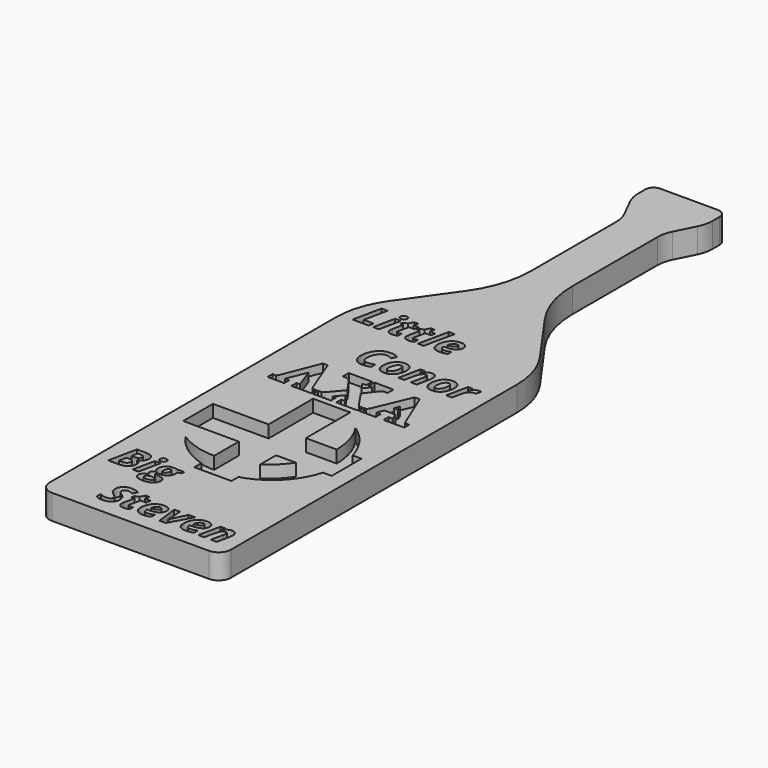
from build123d import *

# Parameters (mm, degrees)
F1_DEPTH     = 19.05
F2_TEXT_SIZE = 30.8680555556
F3_DEPTH     = 6.35
F4_TEXT_SIZE = 30.8680555556
F5_DEPTH     = 6.35
F7_DEPTH     = 6.35
F9_DEPTH     = 9.525


# Not quite as in the source:
# - Text() gives the source's letters only with a copy of the font that has no kerning and outlines rounded to 1/6400 em; it was checked with that copy


with BuildPart() as f1:
    # F0 (on Top) → F1 (new body)
    with BuildSketch(Plane.XY):
        with BuildLine():
            Line((0, 537.45772232), (0, 0))
            Line((0, 0), (60.325, 0))
            ThreePointArc((60.325, 0), (67.0601920908, 2.7898079092), (69.85, 9.525))
            Line((69.85, 9.525), (69.85, 284.5887630252))
            ThreePointArc((69.85, 284.5887630252), (66.8589444377, 303.8479853106), (58.16755455, 321.2928641648))
            Line((58.16755455, 321.2928641648), (29.8939345401, 361.2085630023))
            ThreePointArc((29.8939345401, 361.2085630023), (19.4642666748, 382.1424176272), (15.875, 405.2534843697))
            Line((15.875, 405.2534843697), (15.875, 487.0115956915))
            ThreePointArc((15.875, 487.0115956915), (16.5544756675, 492.8473198735), (18.5565493486, 498.3708210172))
            Line((18.5565493486, 498.3708210172), (25.8934506514, 513.0446236228))
            ThreePointArc((25.8934506514, 513.0446236228), (27.8955243325, 518.5681247666), (28.575, 524.4038489485))
            Line((28.575, 524.4038489485), (28.575, 531.10772232))
            ThreePointArc((28.575, 531.10772232), (26.7151280605, 535.5978503806), (22.225, 537.45772232))
            Line((22.225, 537.45772232), (0, 537.45772232))
        make_face()
        with BuildLine():
            Line((-60.325, 0), (0, 0))
            Line((0, 0), (0, 537.45772232))
            Line((0, 537.45772232), (-22.225, 537.45772232))
            ThreePointArc((-22.225, 537.45772232), (-26.7151280605, 535.5978503806), (-28.575, 531.10772232))
            Line((-28.575, 531.10772232), (-28.575, 524.4038489485))
            ThreePointArc((-28.575, 524.4038489485), (-27.8955243325, 518.5681247666), (-25.8934506514, 513.0446236228))
            Line((-25.8934506514, 513.0446236228), (-18.5565493486, 498.3708210172))
            ThreePointArc((-18.5565493486, 498.3708210172), (-16.5544756675, 492.8473198735), (-15.875, 487.0115956915))
            Line((-15.875, 487.0115956915), (-15.875, 405.2534843697))
            ThreePointArc((-15.875, 405.2534843697), (-19.4642666748, 382.1424176272), (-29.8939345401, 361.2085630023))
            Line((-29.8939345401, 361.2085630023), (-58.16755455, 321.2928641648))
            ThreePointArc((-58.16755455, 321.2928641648), (-66.8589444377, 303.8479853106), (-69.85, 284.5887630252))
            Line((-69.85, 284.5887630252), (-69.85, 9.525))
            ThreePointArc((-69.85, 9.525), (-67.0601920908, 2.7898079092), (-60.325, 0))
        make_face()
    extrude(amount=F1_DEPTH)

    # F2 (on face) → F3 (cut)
    with BuildSketch(Plane.XY.offset(19.05)):
        with Locations((-60.9354709201, 288.925)):
            Text('Little', F2_TEXT_SIZE, font='Open Sans', font_style=FontStyle.BOLDITALIC, text_align=(TextAlign.LEFT, TextAlign.BOTTOM))
        with Locations((-28.8519856771, 246.9444444444)):
            Text('Conor', F2_TEXT_SIZE, font='Open Sans', font_style=FontStyle.BOLDITALIC, text_align=(TextAlign.LEFT, TextAlign.BOTTOM))
    extrude(amount=-F3_DEPTH, mode=Mode.SUBTRACT)

    # F4 (on face) → F5 (cut)
    with BuildSketch(Plane.XY.offset(19.05)):
        with Locations((-61.1838623047, 53.975)):
            Text('Big', F4_TEXT_SIZE, font='Open Sans', font_style=FontStyle.BOLDITALIC, text_align=(TextAlign.LEFT, TextAlign.BOTTOM))
        with Locations((-37.1212483724, 11.9944444444)):
            Text('Steven', F4_TEXT_SIZE, font='Open Sans', font_style=FontStyle.BOLDITALIC, text_align=(TextAlign.LEFT, TextAlign.BOTTOM))
    extrude(amount=-F5_DEPTH, mode=Mode.SUBTRACT)

    # F6 (on face) → F7 (cut)
    with BuildSketch(Plane.XY.offset(19.05)):
        Polygon((-34.6301756799, 233.1359684467), (-38.4192727506, 233.1359684467), (-49.6437177062, 204.600289464), (-50.7918559015, 203.3730298281), (-53.420368582, 203.3730298281), (-53.420368582, 198.6413896084), (-40.5297167599, 198.6413896084), (-40.5297167599, 203.3730298281), (-43.7503643334, 203.3730298281), (-37.7224199474, 218.5051739216), (-32.3315449059, 203.3730298281), (-34.8818972707, 203.3730298281), (-34.8818972707, 198.5394954681), (-19.6526478976, 198.5394954681), (-19.6526478976, 203.6887854338), (-22.0572650433, 203.6887854338), (-23.5543586314, 204.5720219612), align=None)
        Polygon((-18.4506811202, 203.6887854338), (-18.4506811202, 198.5394954681), (-4.4584022835, 198.4982788563), (-4.4584022835, 203.264862299), (-7.0421330656, 203.264862299), (-1.8131635385, 209.4387066198), (2.4278352503, 203.264862299), (-0.3491672687, 203.264862299), (-0.3491672687, 198.4982788563), (16.1199904978, 198.4982788563), (16.1199904978, 203.264862299), (14.0304649249, 203.264862299), (13.2277905941, 203.4942060709), (12.4955335632, 204.126149416), (3.7788371556, 216.8155014515), (10.6649613008, 225.6873100996), (11.4363506436, 226.5358418226), (12.7862812951, 227.4509817362), (15.9875452518, 227.4509817362), (15.9875452518, 233.1359684467), (1.2154448777, 233.1359684467), (1.2154448777, 227.4509817362), (4.1081537493, 227.4509817362), (0, 222.4089205265), (-3.4608505666, 227.4509817362), (-0.4770221421, 227.4509817362), (-0.4770221421, 233.1359684467), (-18.4506811202, 233.1359684467), (-18.4506811202, 227.4509817362), (-15.7873407006, 227.4509817362), (-13.8674285263, 226.7973870039), (-12.5194052234, 225.694462657), (-5.2096643485, 215.1326686144), (-14.0057792887, 204.7470957041), (-15.8274602145, 203.6887854338), align=None)
        Polygon((29.8856571317, 203.264862299), (26.6099330038, 203.264862299), (28.6676567048, 208.4246873856), (37.3272448778, 208.4246873856), (39.142690599, 203.264862299), (36.0063277185, 203.264862299), (36.0063277185, 198.4982788563), (51.921413169, 198.5394954681), (51.906324923, 203.264862299), (49.3972338736, 203.264862299), (48.3452873993, 203.928912447), (47.8699617088, 204.7470957041), (36.1939147115, 233.1359684467), (32.2666428983, 233.1359684467), (20.2097692043, 204.7470957041), (19.3134278219, 203.6887854338), (18.6963006854, 203.264862299), (16.9773567468, 203.264862299), (16.9773567468, 198.4982788563), (29.8856571317, 198.5394954681), align=None)
        Polygon((31.2277458475, 214.315768432), (32.9303331673, 218.3246463537), (34.5791428064, 214.315768432), align=None, mode=Mode.SUBTRACT)
    extrude(amount=-F7_DEPTH, mode=Mode.SUBTRACT)

    # F8 (on face) → F9 (cut)
    with BuildSketch(Plane.XY.offset(19.05)):
        with BuildLine():
            ThreePointArc((-14.3407554962, 98.4615007538), (-29.5492344659, 100.7163979498), (-43.4491820633, 107.2870790958))
            ThreePointArc((-43.4491820633, 107.2870790958), (-30.7685646921, 94.1305929729), (-14.3407554962, 86.1294512392))
            Line((-14.3407554962, 86.1294512392), (-14.3407554962, 79.375))
            Line((-14.3407554962, 79.375), (14.3145304173, 79.375))
            Line((14.3145304173, 79.375), (14.3145304173, 86.1028811304))
            ThreePointArc((14.3145304173, 86.1028811304), (37.075628536, 99.4606450902), (50.4365999476, 122.2198605537))
            Line((50.4365999476, 122.2198605537), (57.15, 122.2198605537))
            Line((57.15, 122.2198605537), (57.15, 150.8768379948))
            Line((57.15, 150.8768379948), (50.4135866296, 150.8768379948))
            ThreePointArc((50.4135866296, 150.8768379948), (42.4067558599, 167.3157610025), (29.2380396277, 180.0016760826))
            ThreePointArc((29.2380396277, 180.0016760826), (35.8168203078, 166.0947605717), (38.0745817448, 150.8768379948))
            Line((38.0745817448, 150.8768379948), (14.3145304173, 150.8768379948))
            Line((14.3145304173, 150.8768379948), (14.3145304173, 193.675))
            Line((14.3145304173, 193.675), (-14.3407554962, 193.675))
            Line((-14.3407554962, 193.675), (-14.3179716542, 150.829538703))
            Line((-14.3179716542, 150.829538703), (-57.15, 150.829538703))
            Line((-57.15, 150.829538703), (-57.15, 122.2198605537))
            Line((-57.15, 122.2198605537), (-14.3407554962, 122.2198605537))
            Line((-14.3407554962, 122.2198605537), (-14.3407554962, 98.4615007538))
        make_face()
        with BuildLine():
            Line((14.3145304173, 106.9878625306), (14.3145304173, 122.2198605537))
            Line((14.3145304173, 122.2198605537), (29.5471155165, 122.2198605537))
            ThreePointArc((29.5471155165, 122.2198605537), (22.721770661, 113.8128833632), (14.3145304173, 106.9878625306))
        make_face(mode=Mode.SUBTRACT)
    extrude(amount=-F9_DEPTH, mode=Mode.SUBTRACT)


solid = f1.part
